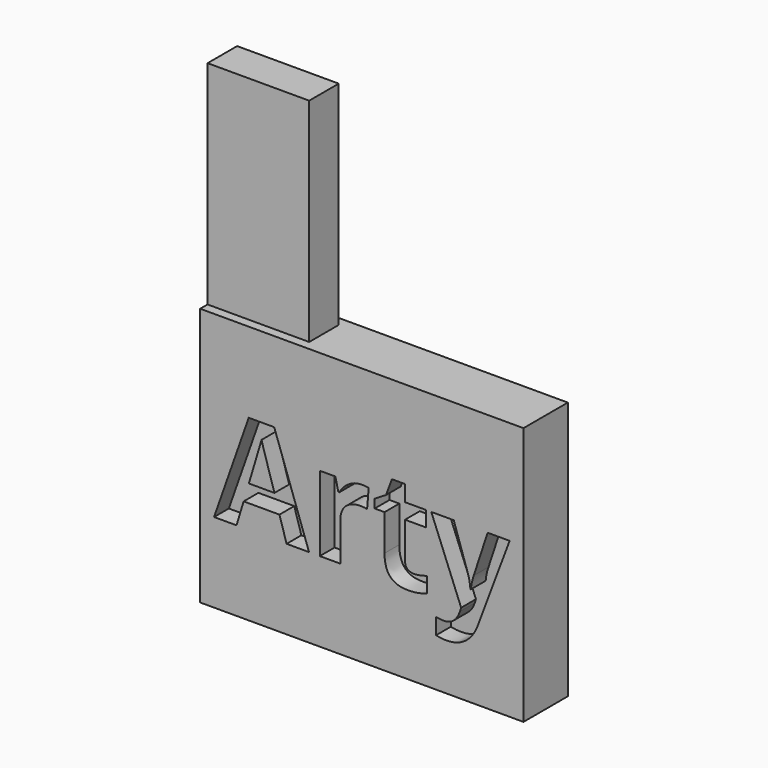
from build123d import *

# Parameters (mm, degrees)
F0_W         = 111.125
F0_H         = 88.9
F1_DEPTH     = 9.525
F2_W         = 34.925
F2_H         = 73.025
F3_DEPTH     = 6.35
F4_TEXT_SIZE = 47.3211556655
F5_DEPTH     = 6.35


# Not quite as in the source:
# - Text() gives the source's letters only with a copy of the font that has no kerning and outlines rounded to 1/6400 em; it was checked with that copy


with BuildPart() as f1:
    # F0 (on Front) → F1 (new body, symmetric)
    with BuildSketch(Plane.XZ):
        Rectangle(F0_W, F0_H)
    extrude(amount=F1_DEPTH, both=True)

    # F2 (on Front) → F3 (join, symmetric)
    with BuildSketch(Plane.XZ):
        with Locations((-38.1, 80.9625)):
            Rectangle(F2_W, F2_H)
    extrude(amount=F3_DEPTH, both=True)

    # F4 (on face) → F5 (cut)
    with BuildSketch(Plane.XZ.offset(9.525)):
        with Locations((-50.8, -17.0356160396)):
            Text('Arty', F4_TEXT_SIZE, font='Open Sans', font_style=FontStyle.BOLD, text_align=(TextAlign.LEFT, TextAlign.BOTTOM))
    extrude(amount=-F5_DEPTH, mode=Mode.SUBTRACT)


solid = f1.part
